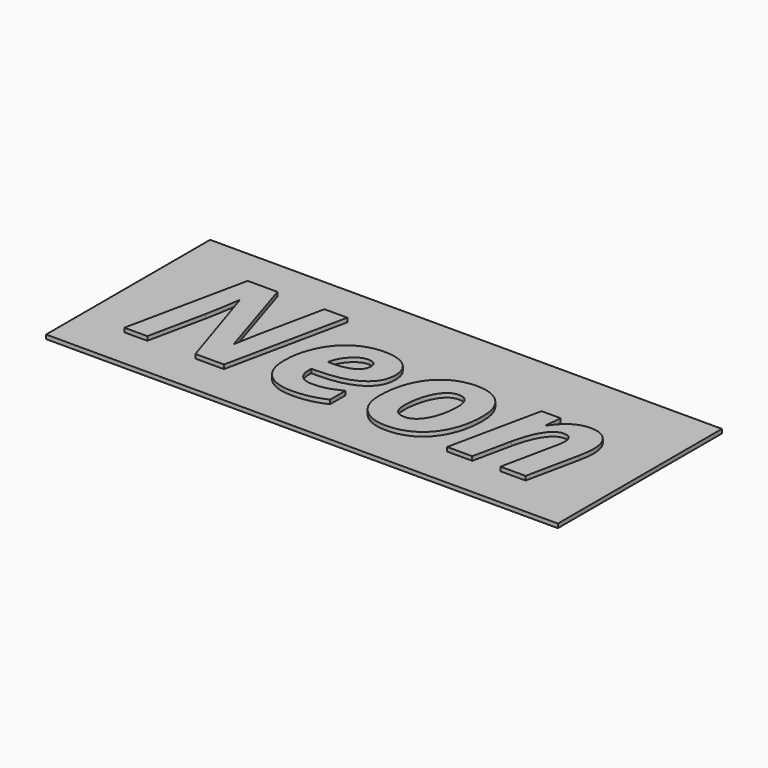
from build123d import *

# Parameters (mm, degrees)
F1_W         = 124.7981770833
F1_H         = 50
F2_DEPTH     = 1
F0_TEXT_SIZE = 41.6666666667
F3_DEPTH     = 1


# Not quite as in the source:
# - Text() gives the source's letters only with a copy of the font that has no kerning and outlines rounded to 1/6400 em; it was checked with that copy


with BuildPart() as f2:
    # F1 (on Top) → F2 (new body)
    with BuildSketch(Plane.XY):
        with Locations((52.3990885417, 15)):
            Rectangle(F1_W, F1_H)
    extrude(amount=-F2_DEPTH)

    # F0 (on Top) → F3 (join)
    with BuildSketch(Plane.XY):
        with Locations((0, 0)):
            Text('Neon', F0_TEXT_SIZE, font='Open Sans', font_style=FontStyle.BOLDITALIC, text_align=(TextAlign.LEFT, TextAlign.BOTTOM))
    extrude(amount=F3_DEPTH)


solid = f2.part
